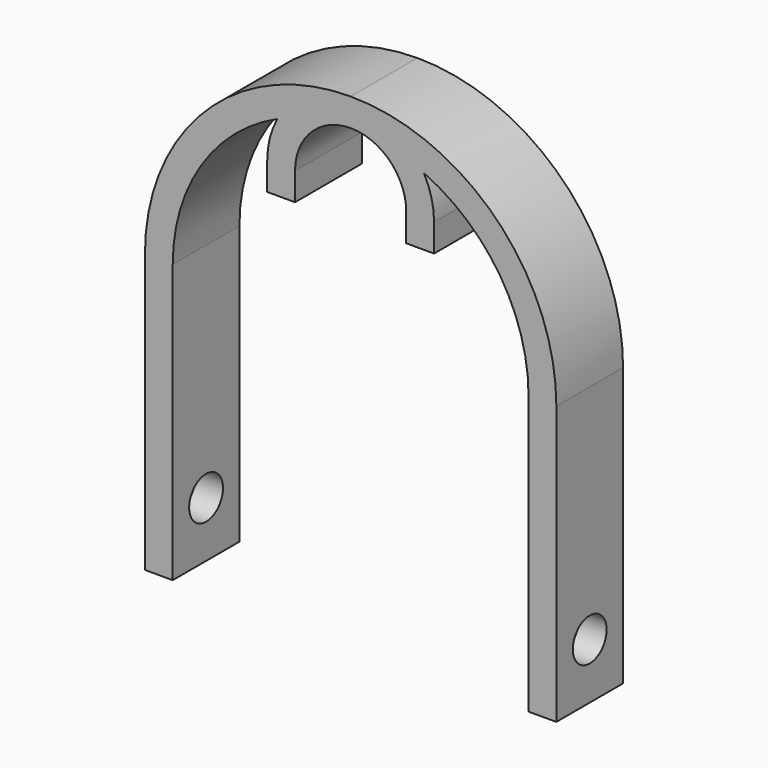
from build123d import *

# Parameters (mm, degrees)
F0_W     = 6.35
F0_H     = 6.35
F1_DEPTH = 19.05
F2_R     = 4.826
F3_DEPTH = 93.9810005078


# Not quite as in the source:
# - ends of sketch curves that miss each other by under 0.0002 mm in the source are joined


with BuildPart() as f1:
    # F0 (on Front) → F1 (new body)
    with BuildSketch(Plane.XZ):
        with BuildLine():
            Line((-40.64, -63.5), (-40.64, 0))
            ThreePointArc((-40.64, 0), (-34.1462652747, 22.0372903913), (-16.7402870182, 37.0320454545))
            ThreePointArc((-16.7402870182, 37.0320454545), (-9.7390716727, 44.3123236883), (0, 46.99))
            ThreePointArc((0, 46.99), (-33.2269478275, 33.2269478275), (-46.9900002539, 0))
            Line((-46.9900002539, 0), (-46.9900002539, -63.5))
            Line((-46.9900002539, -63.5), (-40.64, -63.5))
        make_face()
        with BuildLine():
            ThreePointArc((0, 46.99), (-9.7390716727, 44.3123236883), (-16.7402870182, 37.0320454545))
            ThreePointArc((-16.7402870182, 37.0320454545), (-8.5623382423, 39.727773205), (2.25e-08, 40.64))
            ThreePointArc((2.25e-08, 40.64), (8.5623382643, 39.7277732002), (16.7402870182, 37.0320454545))
            ThreePointArc((16.7402870182, 37.0320454545), (9.7390716727, 44.3123236883), (0, 46.99))
        make_face()
        with BuildLine():
            ThreePointArc((16.7402870182, 37.0320454545), (34.1462652747, 22.0372903913), (40.64, 0))
            Line((40.64, 0), (40.64, -63.5))
            Line((40.64, -63.5), (46.9900002539, -63.5))
            Line((46.9900002539, -63.5), (46.9900002539, 0))
            ThreePointArc((46.9900002539, 0), (33.2269478275, 33.2269478275), (0, 46.9900002539))
            ThreePointArc((0, 46.9900002539), (9.7390716727, 44.3123236883), (16.7402870182, 37.0320454545))
        make_face()
        with BuildLine():
            ThreePointArc((19.05, 27.94), (18.463544726, 32.6304174816), (16.7402870182, 37.0320454545))
            ThreePointArc((16.7402870182, 37.0320454545), (8.5623382643, 39.7277732002), (2.25e-08, 40.64))
            ThreePointArc((2.25e-08, 40.64), (8.980256129, 36.9202561131), (12.7, 27.94))
            Line((12.7, 27.94), (19.05, 27.94))
        make_face()
        with BuildLine():
            ThreePointArc((2.25e-08, 40.64), (-8.5623382423, 39.727773205), (-16.7402870182, 37.0320454545))
            ThreePointArc((-16.7402870182, 37.0320454545), (-18.463544726, 32.6304174816), (-19.05, 27.94))
            Line((-19.05, 27.94), (-12.7, 27.94))
            ThreePointArc((-12.7, 27.94), (-8.9802561131, 36.920256129), (2.25e-08, 40.64))
        make_face()
        with Locations((15.875, 24.765)):
            Rectangle(F0_W, F0_H)
        with Locations((-15.875, 24.765)):
            Rectangle(F0_W, F0_H)
    extrude(amount=-F1_DEPTH)

    # F2 (on face) → F3 (cut, through all)
    with BuildSketch(Plane.YZ.offset(46.9900002539)):
        with Locations((9.525, -50.8)):
            Circle(F2_R)
    extrude(amount=-F3_DEPTH, mode=Mode.SUBTRACT)


solid = f1.part
